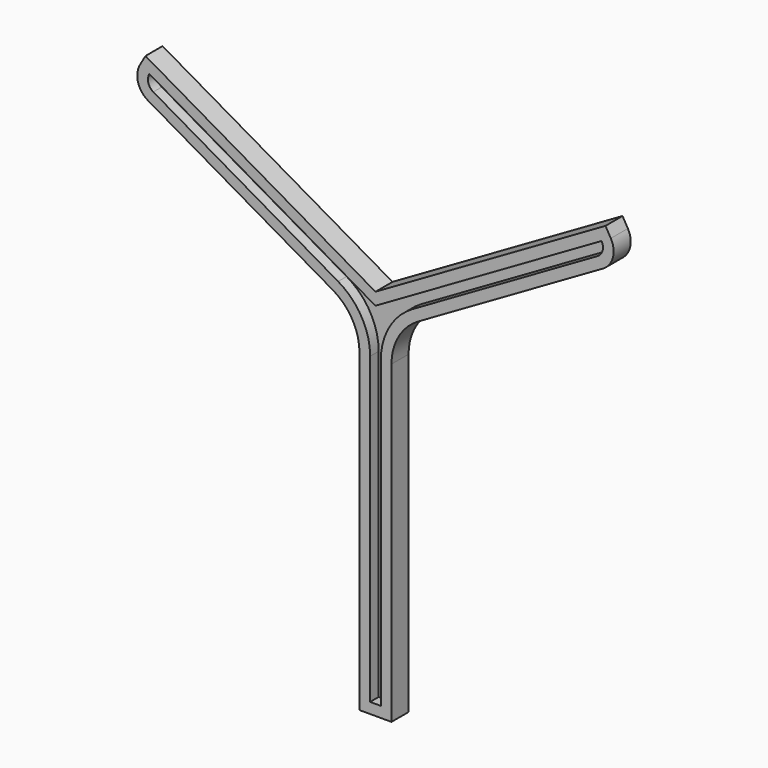
from build123d import *

# Parameters (mm, degrees)
F1_DEPTH    = 1
F2_T        = 1
F2_T3_DEPTH = 4


# Not quite as in the source:
# - a shell that OpenCascade refuses in one call is made with other operations: the cavity is built on its own and cut out


with BuildPart() as f1:
    # F0 (on Front) → F1 (new body, symmetric)
    with BuildSketch(Plane.XZ):
        with BuildLine():
            Line((0, 29.5151724427), (0, 0))
            Line((0, 0), (3, 0))
            Line((3, 0), (3, 29.5151724427))
            ThreePointArc((3, 29.5151724427), (3.6698729811, 32.0151724427), (5.5, 33.8452994616))
            Line((5.5, 33.8452994616), (22.8205080757, 43.8452994616))
            ThreePointArc((22.8205080757, 43.8452994616), (23.7523597283, 45.059712179), (23.5525588833, 46.5773502692))
            Line((23.5525588833, 46.5773502692), (23.0525588833, 47.443375673))
            Line((23.0525588833, 47.443375673), (1.5, 35))
            Line((1.5, 35), (-20.0525588833, 47.443375673))
            Line((-20.0525588833, 47.443375673), (-20.5525588833, 46.5773502692))
            ThreePointArc((-20.5525588833, 46.5773502692), (-20.7523597283, 45.059712179), (-19.8205080757, 43.8452994616))
            Line((-19.8205080757, 43.8452994616), (-2.5, 33.8452994616))
            ThreePointArc((-2.5, 33.8452994616), (-0.6698729811, 32.0151724427), (0, 29.5151724427))
        make_face()
    extrude(amount=F1_DEPTH, both=True)

    # F2: shell of thickness 1, made by hand


with BuildPart() as f2_core1:
    # F2_t2: copy of F1
    add(f1.part)

    # the walls: a layer under each face that stays
    f2_faces = [f2_core1.faces().sort_by_distance(p)[0] for p in [
        (12.2762794416, 0, 41.2216878365),
        (23.3025588833, 0, 47.0103629711),
        (23.7523597283, 0, 45.059712179),
        (14.1602540378, 0, 38.8452994616),
        (3.6698729811, 0, 32.0151724427),
        (3, 0, 14.7575862213),
        (1.5, 0, 0),
        (0, 0, 14.7575862213),
        (-0.6698729811, 0, 32.0151724427),
        (-11.1602540378, 0, 38.8452994616),
        (-20.7523597283, 0, 45.059712179),
        (-20.3025588833, 0, 47.0103629711),
        (-9.2762794416, 0, 41.2216878365),
        (1.5, 1, 23.7216878365),
    ]]
    thicken(f2_faces, amount=-F2_T, mode=Mode.SUBTRACT)

    # F2_s4 → F2_t3 (cut)
    with BuildSketch(Plane.XZ.offset(-2)):
        Polygon((1.5, 35.0173205081), (2, 34.1339745962), (1.5, 33.8452994616), (1, 34.1339745962), align=None)
    extrude(amount=F2_T3_DEPTH, mode=Mode.SUBTRACT)


with BuildPart() as f1_1:
    add(f1.part)

    # what is left inside the walls is the cavity
    f2_cavity = [f2_core1.part.solids().sort_by_distance(p)[0] for p in [
        (1.5, -0.01, 16.025783),
    ]]
    add(f2_cavity, mode=Mode.SUBTRACT)


solid = f1_1.part
